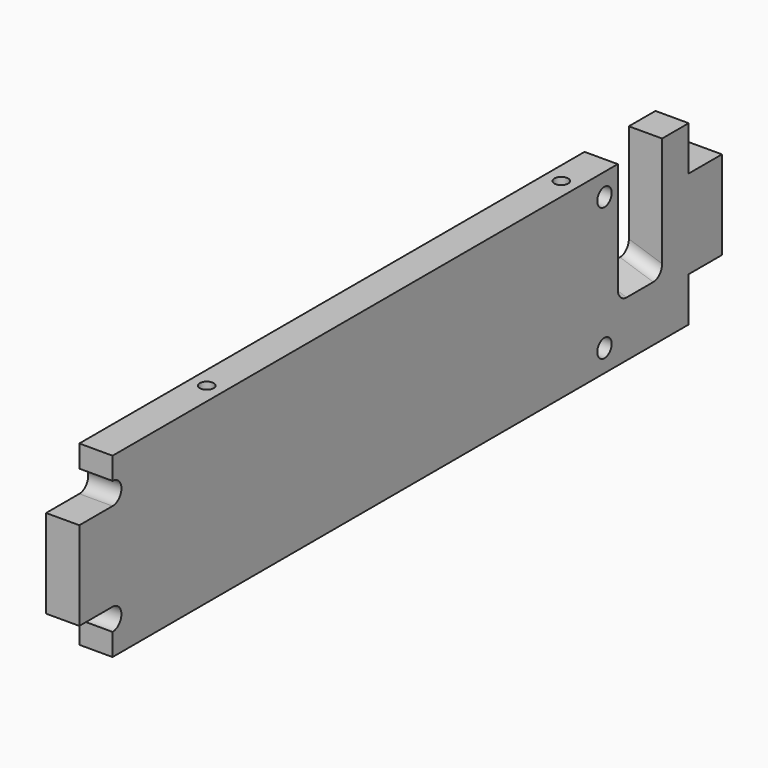
from build123d import *

# Parameters (mm, degrees)
F0_W        = 29.21
F0_H        = 38.1
F0_W_2      = 38.1
F0_W_3      = 25.4
F1_DEPTH    = 9.525
F2_D        = 5.159375
F3_T1_DEPTH = 15.875
F4_R        = 3.175
F6_D        = 3.96875
F6_DEPTH    = 12.7
F6_TIP      = 1.1923327909
F8_D        = 3.96875
F8_DEPTH    = 12.7
F8_TIP      = 1.1923327909
F9_DEPTH    = 6.985
F10_R       = 3.175


# Not quite as in the source:
# - a fillet or chamfer that OpenCascade refuses, or shapes differently, is made with other operations: its cross-section is extruded or revolved along the edge and cut away or added
# - a feature names something its author has since deleted; it is built from what else it names


with BuildPart() as f1:
    # F0 (on Right) → F1 (new body)
    with BuildSketch(Plane.YZ):
        with BuildLine():
            Line((-178.4655057571, -6.35), (-178.4655057571, -12.7))
            Line((-178.4655057571, -12.7), (27.9094942429, -12.7))
            Line((27.9094942429, -12.7), (27.9094942429, 0))
            Line((27.9094942429, 0), (39.8157442429, 0))
            Line((39.8157442429, 0), (39.8157442429, 25.4))
            Line((39.8157442429, 25.4), (27.9094942429, 25.4))
            Line((27.9094942429, 25.4), (27.9094942429, 38.1))
            Line((27.9094942429, 38.1), (18.3844942429, 38.1))
            Line((18.3844942429, 38.1), (18.3844942429, 6.35))
            Line((18.3844942429, 6.35), (2.5094942429, 6.35))
            Line((2.5094942429, 6.35), (2.5094942429, 12.242799294))
            Line((2.5094942429, 12.242799294), (2.5094942429, 38.1))
            Line((2.5094942429, 38.1), (-178.4655057571, 38.1))
            Line((-178.4655057571, 38.1), (-178.4655057571, 31.75))
            ThreePointArc((-178.4655057571, 31.75), (-175.2905057571, 28.575), (-178.4655057571, 25.4))
            Line((-178.4655057571, 25.4), (-190.3717557571, 25.4))
            Line((-190.3717557571, 25.4), (-190.3717557571, 0))
            Line((-190.3717557571, 0), (-178.4655057571, 0))
            ThreePointArc((-178.4655057571, 0), (-175.2905057571, -3.175), (-178.4655057571, -6.35))
        make_face()
        with Locations((-157.5105057571, 12.7)):
            Rectangle(F0_W, F0_H, mode=Mode.SUBTRACT)
        with Locations((-115.6005057571, 12.7)):
            Rectangle(F0_W_2, F0_H, mode=Mode.SUBTRACT)
        with Locations((-69.2455057571, 12.7)):
            Rectangle(F0_W_2, F0_H, mode=Mode.SUBTRACT)
        with Locations((-29.2405057571, 12.7)):
            Rectangle(F0_W_3, F0_H, mode=Mode.SUBTRACT)
        with Locations((-157.5105057571, 12.7)):
            Rectangle(F0_W, F0_H)
        with Locations((-115.6005057571, 12.7)):
            Rectangle(F0_W_2, F0_H)
        with Locations((-69.2455057571, 12.7)):
            Rectangle(F0_W_2, F0_H)
        with Locations((-29.2405057571, 12.7)):
            Rectangle(F0_W_3, F0_H)
    extrude(amount=F1_DEPTH)

    # F2 (through all)
    with Locations(Plane(origin=(0, 0, 0), x_dir=(0, 1, 0), z_dir=(-1, 0, 0))):
        with Locations((-2.2530057571, -31.75), (-2.2530057571, 6.35)):
            Hole(F2_D / 2)

    # F3: chamfer of 3.175 x 9.525 on 1 edges, made by hand

    # F3_s2 → F3_t1 (cut)
    with BuildSketch(Plane.XZ.offset(-18.3844942429)):
        Polygon((0, 6.35), (9.525, 3.175), (9.525, 6.35), align=None)
    extrude(amount=F3_T1_DEPTH, mode=Mode.SUBTRACT)

    # F4
    f4_edges = [f1.edges().sort_by_distance(p)[0] for p in [
        (4.7625, 18.384494, 4.7625),
        (4.7625, 2.509494, 4.7625),
    ]]
    fillet(f4_edges, radius=F4_R)

    # F6
    with Locations(Plane.XY.offset(38.1)):
        with Locations((4.7625, -138.7780057571), (4.7625, -11.7780057571)):
            Hole(F6_D / 2, depth=F6_DEPTH)
            with Locations((0, 0, -(F6_DEPTH + F6_TIP / 2))):  # 118° drill point
                Cone(0, F6_D / 2, F6_TIP, mode=Mode.SUBTRACT)

    # F8
    with Locations(Plane(origin=(0, 0, -12.7), x_dir=(1, 0, 0), z_dir=(0, 0, -1))):
        with Locations((4.7625, 138.7780057571), (4.7625, 11.7780057571)):
            Hole(F8_D / 2, depth=F8_DEPTH)
            with Locations((0, 0, -(F8_DEPTH + F8_TIP / 2))):  # 118° drill point
                Cone(0, F8_D / 2, F8_TIP, mode=Mode.SUBTRACT)

    # F0 (on Right) → F9 (cut)
    with BuildSketch(Plane.YZ):
        with Locations((-29.2405057571, 12.7)):
            Rectangle(F0_W_3, F0_H)
        with Locations((-69.2455057571, 12.7)):
            Rectangle(F0_W_2, F0_H)
        with Locations((-115.6005057571, 12.7)):
            Rectangle(F0_W_2, F0_H)
        with Locations((-157.5105057571, 12.7)):
            Rectangle(F0_W, F0_H)
    extrude(amount=F9_DEPTH, mode=Mode.SUBTRACT)

    # F10
    f10_edges = [f1.edges().sort_by_distance(p)[0] for p in [
        (3.4925, -16.540506, 31.75),
        (3.4925, -50.195506, 31.75),
        (3.4925, -96.550506, 31.75),
        (3.4925, -142.905506, 31.75),
        (3.4925, -172.115506, 31.75),
        (3.4925, -134.650506, 31.75),
        (3.4925, -88.295506, 31.75),
        (3.4925, -41.940506, 31.75),
        (3.4925, -16.540506, -6.35),
        (3.4925, -50.195506, -6.35),
        (3.4925, -96.550506, -6.35),
        (3.4925, -142.905506, -6.35),
        (3.4925, -41.940506, -6.35),
        (3.4925, -88.295506, -6.35),
        (3.4925, -134.650506, -6.35),
        (3.4925, -172.115506, -6.35),
    ]]
    fillet(f10_edges, radius=F10_R)


solid = f1.part
